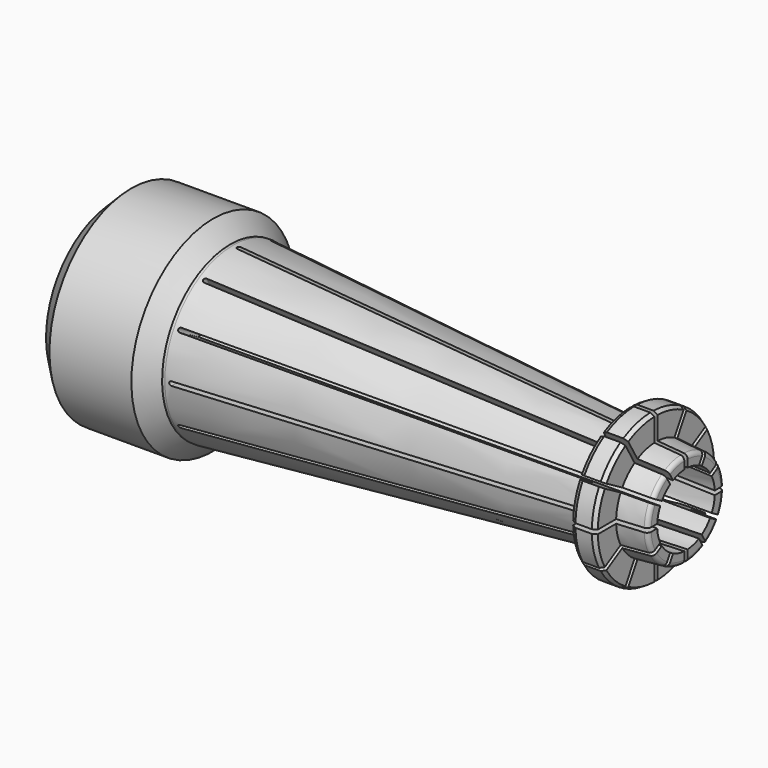
from build123d import *

# Parameters (mm, degrees)
F2_C1_SIZE2     = 0.762
F2_C1_SIZE      = 0.4399409051
F2_C2_SIZE2     = 0.4399409051
F2_C2_SIZE      = 0.762
F3_R            = 0.762
F4_SIZE2        = 1.524
F4_SIZE         = 1.524
F6_DEPTH        = 24.892
F6_COPIES_COUNT = 6
F6_COPIES_ANGLE = 150


# Not quite as in the source:
# - a pattern or mirror of a feature is missing from the dataset's text; its kind, count and spacing are read off the source's solid


with BuildPart() as f1:
    # F0 (on Front) → F1 (revolve)
    with BuildSketch(Plane.XZ):
        Polygon((18.415, 19.05), (3.175, 19.05), (0, 15.875), (0, 10.16), (22.098, 10.16), (106.3498, 6.7024533834), (106.3498, 8.8017625296), (100.7618, 9.271), (100.7618, 13.97), (96.1898, 13.97), (96.1898, 9.6533377221), (22.098, 15.875), (21.59, 15.875), (18.5293, 18.9357), align=None)
    revolve(axis=Axis((53.1749, 0, 0), (1, 0, 0)))

    # F2: chamfer of 0.762 x 0.4399409051 on 2 edges, made by hand

    # F2_c1
    f2_c1_edges = [f1.edges().sort_by_distance(p)[0] for p in [
        (100.7618, 0, -13.97),
    ]]
    f2_c1_side = f1.faces().sort_by_distance((100.7618, 0, -13.9612011819))[0]
    chamfer(f2_c1_edges, length=F2_C1_SIZE, length2=F2_C1_SIZE2, reference=f2_c1_side)

    # F2_c2
    f2_c2_edges = [f1.edges().sort_by_distance(p)[0] for p in [
        (96.1898, 0, -13.97),
    ]]
    f2_c2_side = f1.faces().sort_by_distance((96.1985988181, 0, -13.97))[0]
    chamfer(f2_c2_edges, length=F2_C2_SIZE, length2=F2_C2_SIZE2, reference=f2_c2_side)

    # F3
    f3_edges = [f1.edges().sort_by_distance(p)[0] for p in [
        (106.3498, 0, -8.801763),
    ]]
    fillet(f3_edges, radius=F3_R)

    # F4
    f4_edges = [f1.edges().sort_by_distance(p)[0] for p in [
        (0, 0, -10.16),
    ]]
    chamfer(f4_edges, length=F4_SIZE, length2=F4_SIZE2)

    # F5 (on Front) → F6 (cut, symmetric)
    with BuildSketch(Plane.XZ):
        with BuildLine():
            Line((107.3643043638, 0.381), (23.241, 0.381))
            ThreePointArc((23.241, 0.381), (22.86, 0), (23.241, -0.381))
            Line((23.241, -0.381), (107.3643043638, -0.381))
            Line((107.3643043638, -0.381), (107.3643043638, 0.381))
        make_face()
    f6 = extrude(amount=F6_DEPTH, both=True, mode=Mode.SUBTRACT)

    # F6_copies: F6 ×6 about axis
    f6_copies_axis = Axis((0, 0, 0), (-1, 0, 0))
    for i in range(1, F6_COPIES_COUNT):
        add(f6.rotate(f6_copies_axis, i * F6_COPIES_ANGLE / (F6_COPIES_COUNT - 1)), mode=Mode.SUBTRACT)


solid = f1.part
